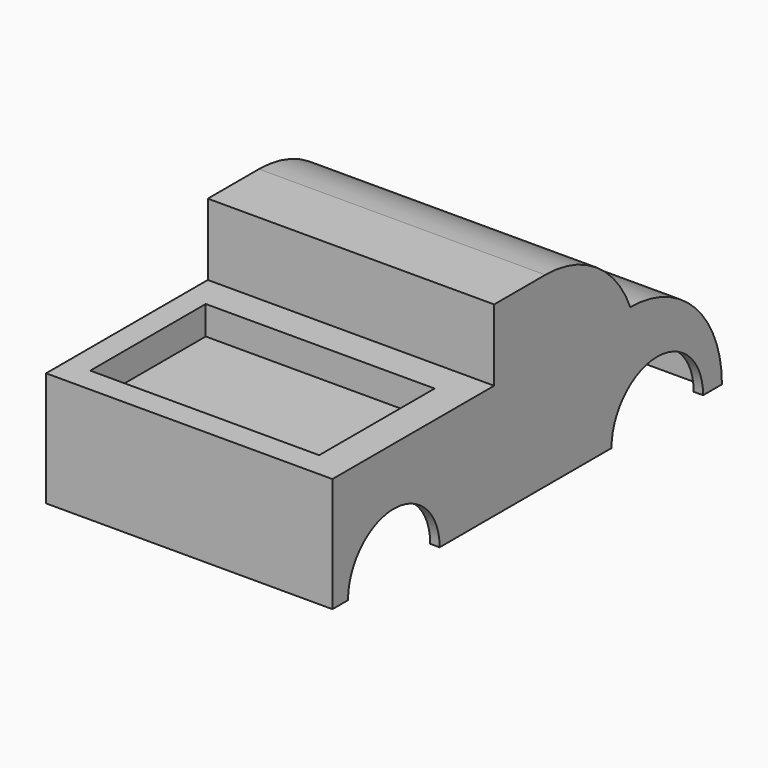
from build123d import *

# Parameters (mm, degrees)
F0_W        = 100
F0_H        = 170
F1_DEPTH    = 40
F2_R        = 39.99999
F3_W        = 100
F3_H        = 59.416816481
F4_DEPTH    = 25
F5_T1_DEPTH = 285.4049621774
F7_DEPTH    = 25
F8_W        = 93.7445983291
F8_H        = 163.0899235606
F9_DEPTH    = 25
F11_DEPTH   = 25
F12_W       = 79.9397490919
F12_H       = 50.4037756473
F13_DEPTH   = 10


# Not quite as in the source:
# - a fillet or chamfer that OpenCascade refuses, or shapes differently, is made with other operations: its cross-section is extruded or revolved along the edge and cut away or added
# - a fillet or chamfer is up to 0.001 mm smaller than in the source, because OpenCascade refuses the exact size


with BuildPart() as f1:
    # F0 (on Top) → F1 (new body)
    with BuildSketch(Plane.XY):
        with Locations((0, 3.7849953254)):
            Rectangle(F0_W, F0_H)
    extrude(amount=F1_DEPTH)

    # F2 (radius 40 in the source; OpenCascade refuses exactly that, so slightly less here)
    f2_edges = [f1.edges().sort_by_distance(p)[0] for p in [
        (0, 88.784995, 40),
    ]]
    fillet(f2_edges, radius=F2_R)

    # F3 (on face) → F4 (join)
    with BuildSketch(Plane.XY.offset(40)):
        with Locations((0, 19.0765870849)):
            Rectangle(F3_W, F3_H)
    extrude(amount=F4_DEPTH)

    # F5: fillet of radius 40 on 1 edges, made by hand

    # F5_s2 → F5_t1 (cut)
    with BuildSketch(Plane.YZ.offset(-142.7024810887)):
        with BuildLine():
            ThreePointArc((48.7849953254, 40), (34.0646826649, 58.1662479036), (11.7040028899, 65))
            Line((11.7040028899, 65), (48.7849953254, 65))
            Line((48.7849953254, 65), (48.7849953254, 40))
        make_face()
    extrude(amount=F5_T1_DEPTH, mode=Mode.SUBTRACT)

    # F6 (on face) → F7 (cut)
    with BuildSketch(Plane.YZ.offset(50)):
        with BuildLine():
            Line((-74.4276870787, 0), (-34.4276870787, 0))
            ThreePointArc((-34.4276870787, 0), (-54.4276870787, 20), (-74.4276870787, 0))
        make_face()
        with BuildLine():
            ThreePointArc((80.5723129213, 0), (60.5723129213, 20), (40.5723129213, 0))
            Line((40.5723129213, 0), (80.5723129213, 0))
        make_face()
    extrude(amount=-F7_DEPTH, mode=Mode.SUBTRACT)

    # F8 (on face) → F9 (cut)
    with BuildSketch(Plane(origin=(0, 0, 0), x_dir=(1, 0, 0), z_dir=(0, 0, -1))):
        with Locations((-0.160522759, -3.6244727671)):
            Rectangle(F8_W, F8_H)
    extrude(amount=-F9_DEPTH, mode=Mode.SUBTRACT)

    # F10 (on face) → F11 (cut)
    with BuildSketch(Plane(origin=(-50, 0, 0), x_dir=(0, -1, 0), z_dir=(-1, 0, 0))):
        with BuildLine():
            ThreePointArc((-77.0112355053, 0), (-57.0112355053, -20), (-37.0112355053, 0))
            Line((-37.0112355053, 0), (-77.0112355053, 0))
        make_face()
        with BuildLine():
            ThreePointArc((77.9887644947, 0), (57.9887644947, 20), (37.9887644947, 0))
            Line((37.9887644947, 0), (77.9887644947, 0))
        make_face()
        with BuildLine():
            Line((-77.0112355053, 0), (-37.0112355053, 0))
            ThreePointArc((-37.0112355053, 0), (-57.0112355053, 20), (-77.0112355053, 0))
        make_face()
        with BuildLine():
            Line((77.9887644947, 0), (37.9887644947, 0))
            ThreePointArc((37.9887644947, 0), (57.9887644947, -20), (77.9887644947, 0))
        make_face()
    extrude(amount=-F11_DEPTH, mode=Mode.SUBTRACT)

    # F12 (on face) → F13 (cut)
    with BuildSketch(Plane.XY.offset(40)):
        with Locations((-1.6052145511, -47.2608646378)):
            Rectangle(F12_W, F12_H)
    extrude(amount=-F13_DEPTH, mode=Mode.SUBTRACT)


solid = f1.part
